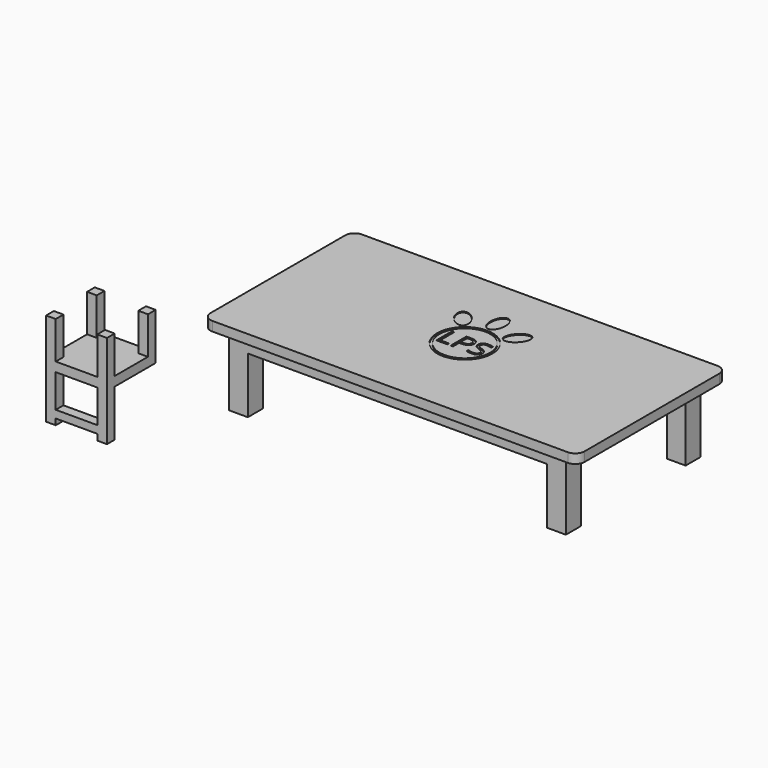
from build123d import *

# Parameters (mm, degrees)
F1_W           = 80
F1_H           = 40
F3_DEPTH       = 2
F4_W           = 2
F4_H           = 2
F6_DEPTH       = 15
F4_H_2         = 28
F4_W_2         = 64
F7_DEPTH       = 3
F8_R           = 2
F9_TEXT_SIZE   = 9.0390692583
F11_DEPTH      = 0.2
F12_R          = 5.9131620378
F12_R_2        = 5.4131620378
F12_TEXT_SIZE  = 5.9027777778
F13_DEPTH      = 0.2
F14_W          = 2.0646750927
F14_H          = 2.0646750927
F15_DEPTH      = 10
F15_DEPTH_BACK = 10
F16_DEPTH      = 10
F17_DEPTH      = 2
F18_W          = 2.0646750927
F18_H          = 1.6348403879
F19_DEPTH      = 8.8873319328


# Not quite as in the source:
# - a feature names something its author has since deleted; it is built from what else it names
# - Text() gives the source's letters only with a copy of the font that has no kerning and outlines rounded to 1/6400 em; it was checked with that copy


with BuildPart() as f3:
    # F1 (on Top) → F3 (new body)
    with BuildSketch(Plane.XY):
        Rectangle(F1_W, F1_H)
    extrude(amount=F3_DEPTH)

    # F4 (on face) → F6 (join)
    with BuildSketch(Plane(origin=(0, 0, 0), x_dir=(1, 0, 0), z_dir=(0, 0, -1))):
        Polygon((-36, 18), (-36, 14), (-34, 14), (-34, 16), (-32, 16), (-32, 18), align=None)
        Polygon((-36, -14), (-36, -18), (-32, -18), (-32, -16), (-34, -16), (-34, -14), align=None)
        Polygon((32, -16), (32, -18), (36, -18), (36, -14), (34, -14), (34, -16), align=None)
        with Locations((-33, 15)):
            Rectangle(F4_W, F4_H)
        with Locations((-33, -15)):
            Rectangle(F4_W, F4_H)
        with Locations((33, -15)):
            Rectangle(F4_W, F4_H)
        with Locations((33, 15)):
            Rectangle(F4_W, F4_H)
        Polygon((34, 14), (36, 14), (36, 18), (32, 18), (32, 16), (34, 16), align=None)
    extrude(amount=F6_DEPTH)

    # F4 (on face) → F7 (join)
    with BuildSketch(Plane(origin=(0, 0, 0), x_dir=(1, 0, 0), z_dir=(0, 0, -1))):
        with Locations((-35, 0)):
            Rectangle(F4_W, F4_H_2)
        with Locations((0, 17)):
            Rectangle(F4_W_2, F4_H)
        with Locations((35, 0)):
            Rectangle(F4_W, F4_H_2)
        with Locations((0, -17)):
            Rectangle(F4_W_2, F4_H)
        Polygon((34, 14), (36, 14), (36, 18), (32, 18), (32, 16), (34, 16), align=None)
        Polygon((-36, 18), (-36, 14), (-34, 14), (-34, 16), (-32, 16), (-32, 18), align=None)
        Polygon((-36, -14), (-36, -18), (-32, -18), (-32, -16), (-34, -16), (-34, -14), align=None)
        Polygon((32, -16), (32, -18), (36, -18), (36, -14), (34, -14), (34, -16), align=None)
    extrude(amount=F7_DEPTH)

    # F8
    f8_edges = [f3.edges().sort_by_distance(p)[0] for p in [
        (-40, -20, 1),
        (40, -20, 1),
        (40, 20, 1),
        (-40, 20, 1),
    ]]
    fillet(f8_edges, radius=F8_R)

    # F9 (on face) → F11 (join)
    with BuildSketch(Plane(origin=(0, 0, 0), x_dir=(1, 0, 0), z_dir=(0, 0, -1))):
        with Locations((-13.3333333333, -3.254064933)):
            Text('Lucka', F9_TEXT_SIZE, font='Open Sans', font_style=FontStyle.BOLD, text_align=(TextAlign.LEFT, TextAlign.BOTTOM))
    extrude(amount=F11_DEPTH)

    # F12 (on face) → F13 (cut)
    with BuildSketch(Plane.XY.offset(2)):
        Circle(F12_R)
        Circle(F12_R_2, mode=Mode.SUBTRACT)
        with BuildLine():
            add(Edge.make_bspline(
                [(4.0147238493, 5.1192573279), (5.9375709184, 3.3754260534), (7.4941608852, 7.0238459042), (9.0507508521, 10.672265755), (5.5713138161, 8.7676771787), (2.0918767801, 6.8630886023), (4.0147238493, 5.1192573279)],
                knots=[0, 0, 0, 2.0943951024, 2.0943951024, 4.1887902048, 4.1887902048, 6.2831853072, 6.2831853072, 6.2831853072], degree=2, weights=[1, 0.5, 1, 0.5, 1, 0.5, 1]))
        make_face()
        with BuildLine():
            add(Edge.make_bspline(
                [(-0.2151382858, 6.5021933755), (2.3787611632, 6.4023233894), (1.2260191824, 10.1977318863), (0.0732772016, 13.9931403832), (-1.3678802665, 10.2976018724), (-2.8090377347, 6.6020633617), (-0.2151382858, 6.5021933755)],
                knots=[0, 0, 0, 2.0943951024, 2.0943951024, 4.1887902048, 4.1887902048, 6.2831853072, 6.2831853072, 6.2831853072], degree=2, weights=[1, 0.5, 1, 0.5, 1, 0.5, 1]))
        make_face()
        with BuildLine():
            add(Edge.make_bspline(
                [(-4.3443348259, 4.8426808789), (-2.2930973773, 6.4335024576), (-5.6157905216, 8.5999857836), (-8.9384836658, 10.7664691096), (-7.6670279701, 7.009164205), (-6.3955722744, 3.2518593003), (-4.3443348259, 4.8426808789)],
                knots=[0, 0, 0, 2.0943951024, 2.0943951024, 4.1887902048, 4.1887902048, 6.2831853072, 6.2831853072, 6.2831853072], degree=2, weights=[1, 0.5, 1, 0.5, 1, 0.5, 1]))
        make_face()
        with Locations((-4.9786241319, -2.125)):
            Text('LPS', F12_TEXT_SIZE, font='Open Sans', text_align=(TextAlign.LEFT, TextAlign.BOTTOM))
    extrude(amount=-F13_DEPTH, mode=Mode.SUBTRACT)


with BuildPart() as f15:
    # F14 (on Top) → F15 (new body, two sides)
    with BuildSketch(Plane.XY) as f15_sk:
        with Locations((-50.2547770739, -46.7736534774)):
            Rectangle(F14_W, F14_H)
    extrude(amount=F15_DEPTH)
    extrude(f15_sk.sketch, amount=-F15_DEPTH_BACK)



with BuildPart() as f15b:
    # F14 (on Top) → F15, piece 2 (new body, two sides)
    with BuildSketch(Plane.XY) as f15_2_sk:
        with Locations((-39.3027700484, -46.7736534774)):
            Rectangle(F14_W, F14_H)
    extrude(amount=F15_DEPTH)
    extrude(f15_2_sk.sketch, amount=-F15_DEPTH_BACK)


with BuildPart() as f16:
    # F14 (on Top) → F16 (new body)
    with BuildSketch(Plane.XY):
        with Locations((-50.2547770739, -35.821646452)):
            Rectangle(F14_W, F14_H)
    extrude(amount=F16_DEPTH)


with BuildPart() as f16b:
    # F14 (on Top) → F16, piece 2 (new body)
    with BuildSketch(Plane.XY):
        with Locations((-39.3027700484, -35.821646452)):
            Rectangle(F14_W, F14_H)
    extrude(amount=F16_DEPTH)


with BuildPart() as f15_1:
    add(f15.part)

    add(f15b.part)  # F17 merges F15b

    add(f16.part)  # F17 merges F16

    add(f16b.part)  # F17 merges F16b
    # F14 (on Top) → F17 (join)
    with BuildSketch(Plane.XY):
        Polygon((-40.3351075947, -34.7893089056), (-49.2224395275, -34.7893089056), (-49.2224395275, -36.8539839983), (-51.2871146202, -36.8539839983), (-51.2871146202, -45.7413159311), (-49.2224395275, -45.7413159311), (-49.2224395275, -47.8059910238), (-40.3351075947, -47.8059910238), (-40.3351075947, -45.7413159311), (-38.270432502, -45.7413159311), (-38.270432502, -36.8539839983), (-40.3351075947, -36.8539839983), align=None)
        with Locations((-50.2547770739, -35.821646452)):
            Rectangle(F14_W, F14_H)
        with Locations((-39.3027700484, -35.821646452)):
            Rectangle(F14_W, F14_H)
    extrude(amount=F17_DEPTH)

    # F18 (on face) → F19 (join, through all)
    with BuildSketch(Plane(origin=(-40.3351075947, 0, 0), x_dir=(0, -1, 0), z_dir=(-1, 0, 0))):
        with Locations((46.7736534774, -7.8962601256)):
            Rectangle(F18_W, F18_H)
    extrude(amount=F19_DEPTH)


solid = Compound([f3.part, f15_1.part])
